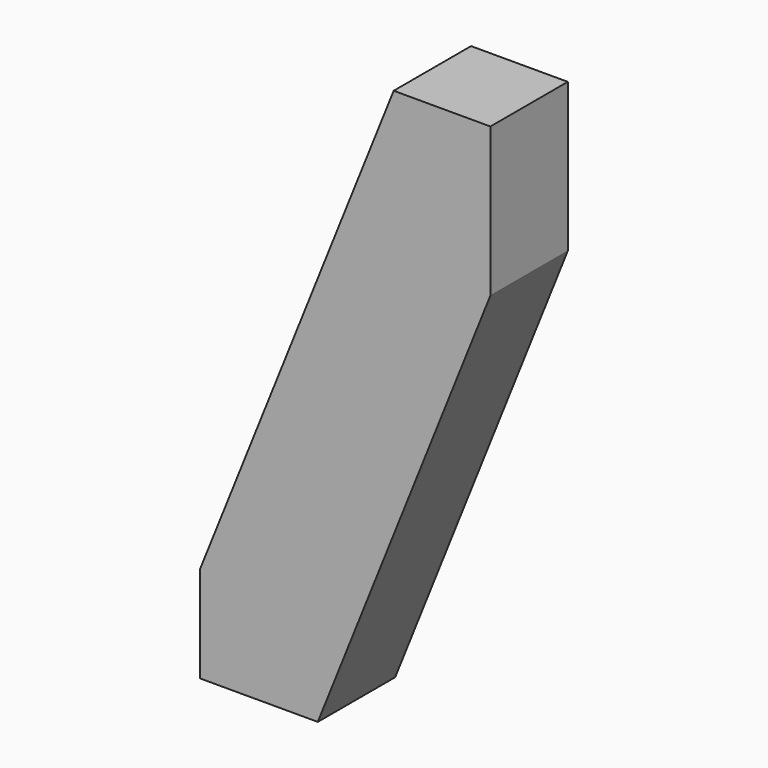
from build123d import *

# Parameters (mm, degrees)
F1_DEPTH = 10
F2_R     = 4.25
F3_DEPTH = 25


with BuildPart() as f1:
    # F0 (on Front) → F1 (new body, symmetric)
    with BuildSketch(Plane.XZ):
        Polygon((-60, 20), (-60, 0), (-35.6890111572, 0), (0, 89.222527893), (0, 120), (-20, 120), align=None)
    extrude(amount=F1_DEPTH, both=True)

    # F2 (on face) → F3 (cut)
    with BuildSketch(Plane(origin=(0, 0, 0), x_dir=(1, 0, 0), z_dir=(0, 0, -1))):
        with Locations((-49, 0)):
            Circle(F2_R)
    extrude(amount=-F3_DEPTH, mode=Mode.SUBTRACT)


solid = f1.part
